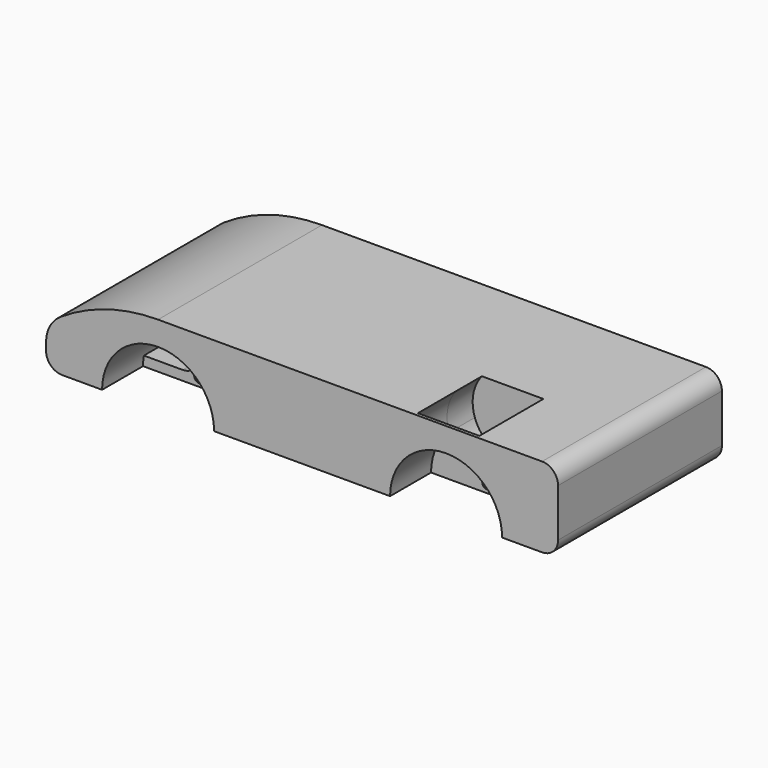
from build123d import *

# Parameters (mm, degrees)
F1_DEPTH      = 64
F2_R          = 5
F3_R          = 10
F5_R          = 1.5
F6_DEPTH      = 32
F7_R          = 5
F9_DEPTH      = 10
F9_DEPTH_BACK = 15


with BuildPart() as f1:
    # F0 (on Front) → F1 (new body)
    with BuildSketch(Plane.XZ):
        with BuildLine():
            Line((0, 12.5), (0, 0))
            Line((0, 0), (17.5, 0))
            ThreePointArc((17.5, 0), (35, 17.5), (52.5, 0))
            Line((52.5, 0), (107.5, 0))
            ThreePointArc((107.5, 0), (125, 17.5), (142.5, 0))
            Line((142.5, 0), (160, 0))
            Line((160, 0), (160, 25))
            Line((160, 25), (35, 25))
            ThreePointArc((35, 25), (16.4174140659, 21.7812406156), (0, 12.5))
        make_face()
    extrude(amount=-F1_DEPTH)

    # F2
    f2_edges = [f1.edges().sort_by_distance(p)[0] for p in [
        (160, 32, 25),
        (0, 32, 0),
        (160, 32, 0),
    ]]
    fillet(f2_edges, radius=F2_R)

    # F3
    f3_edges = [f1.edges().sort_by_distance(p)[0] for p in [
        (0, 32, 12.5),
    ]]
    fillet(f3_edges, radius=F3_R)

    # F5 (on offset) → F6 (join)
    with BuildSketch(Plane.XZ.offset(-16)):
        with BuildLine():
            Line((17.5, 0), (52.5, 0))
            ThreePointArc((52.5, 0), (52.4351146235, 1.5055823014), (52.2409396496, 3))
            Line((52.2409396496, 3), (37.4494897428, 3))
            ThreePointArc((37.4494897428, 3), (35, 5), (32.5505102572, 3))
            Line((32.5505102572, 3), (17.7590603504, 3))
            ThreePointArc((17.7590603504, 3), (17.5648853765, 1.5055823014), (17.5, 0))
        make_face()
        with Locations((35, 2.5)):
            Circle(F5_R, mode=Mode.SUBTRACT)
        with BuildLine():
            Line((107.5, 0), (142.5, 0))
            ThreePointArc((142.5, 0), (125, 17.5), (107.5, 0))
        make_face()
        with Locations((125, 2.5)):
            Circle(F5_R, mode=Mode.SUBTRACT)
    extrude(amount=-F6_DEPTH)

    # F7
    f7_edges = [f1.edges().sort_by_distance(p)[0] for p in [
        (37.44949, 32, 3),
        (32.55051, 32, 3),
    ]]
    fillet(f7_edges, radius=F7_R)

    # F8 (on offset) → F9 (cut, two sides)
    with BuildSketch(Plane.XZ.offset(-16)) as f9_sk:
        with BuildLine():
            ThreePointArc((113.1874502253, 12.9117647059), (125, 4.5), (136.8125497747, 12.9117647059))
            ThreePointArc((136.8125497747, 12.9117647059), (125, 17.5), (113.1874502253, 12.9117647059))
        make_face()
        with BuildLine():
            ThreePointArc((113.1874502253, 12.9117647059), (125, 17.5), (136.8125497747, 12.9117647059))
            ThreePointArc((136.8125497747, 12.9117647059), (137.3269394455, 14.9271845456), (137.5, 17))
            ThreePointArc((137.5, 17), (122.9271845456, 29.3269394455), (113.1874502253, 12.9117647059))
        make_face()
    extrude(amount=-F9_DEPTH, mode=Mode.SUBTRACT)
    extrude(f9_sk.sketch, amount=F9_DEPTH_BACK, mode=Mode.SUBTRACT)


solid = f1.part
